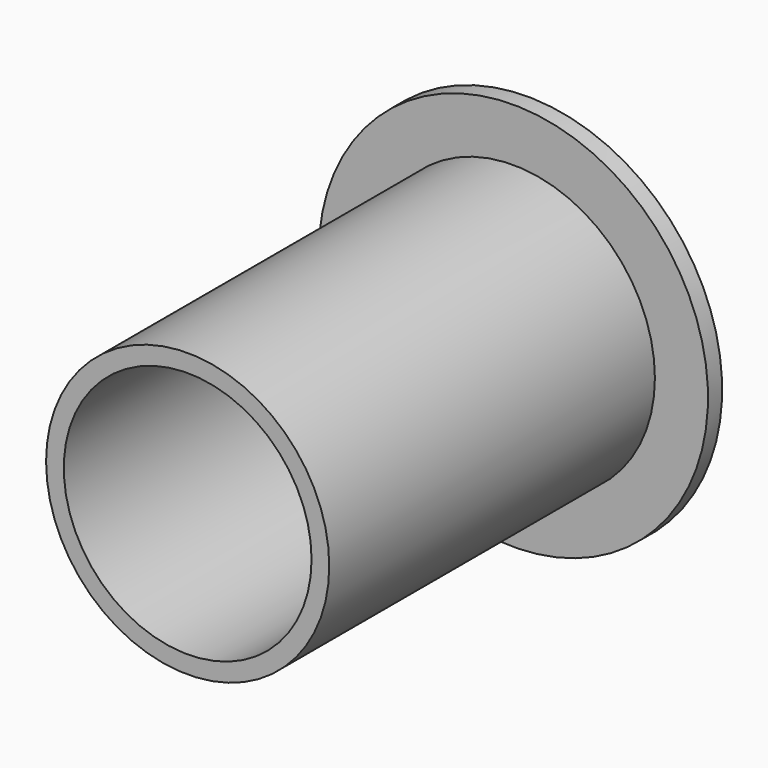
from build123d import *

# Parameters (mm, degrees)
F0_R     = 40
F0_R_2   = 35
F1_DEPTH = 120
F2_R     = 55
F2_R_2   = 40
F2_R_3   = 35
F3_DEPTH = 5


with BuildPart() as f1:
    # F0 (on Front) → F1 (new body)
    with BuildSketch(Plane.XZ):
        Circle(F0_R)
        Circle(F0_R_2, mode=Mode.SUBTRACT)
    extrude(amount=F1_DEPTH)

    # F2 (on face) → F3 (join)
    with BuildSketch(Plane(origin=(0, 0, 0), x_dir=(-1, 0, 0), z_dir=(0, 1, 0))):
        Circle(F2_R)
        Circle(F2_R_2, mode=Mode.SUBTRACT)
        Circle(F2_R_2)
        Circle(F2_R_3, mode=Mode.SUBTRACT)
        Circle(F2_R_3)
    extrude(amount=-F3_DEPTH)


solid = f1.part
